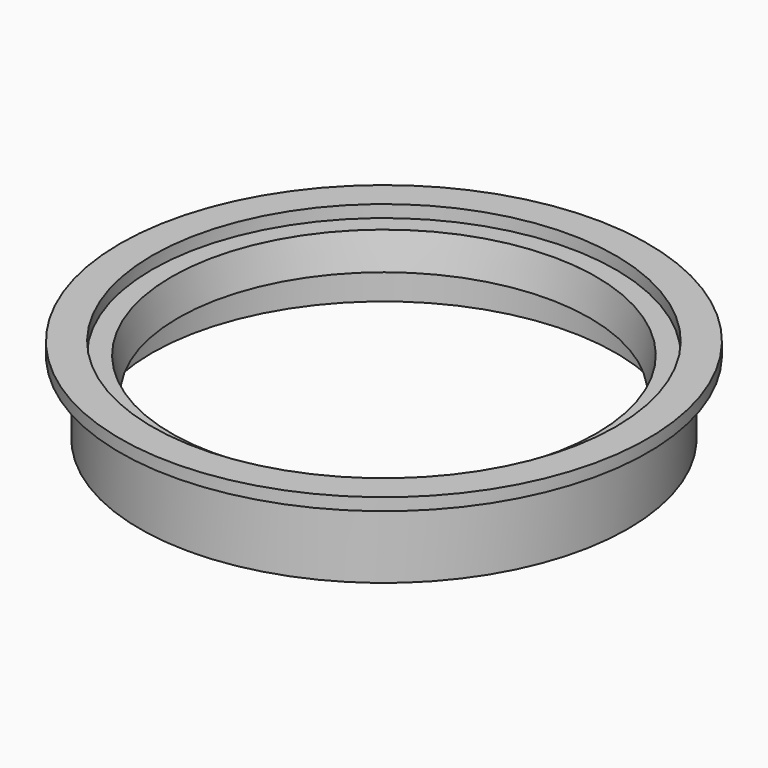
from build123d import *

# Parameters (mm, degrees)
F0_W = 1.2508329971
F0_H = 1.489882911


# Not quite as in the source:
# - ends of sketch curves that miss each other by under 0.0002 mm in the source are joined


with BuildPart() as f1:
    # F0 (on Front) → F1 (revolve)
    with BuildSketch(Plane.XZ):
        Polygon((-10.2681356725, 15.1391583099), (-10.2681356725, 15.1379262976), (-10.2489686697, 15.1379262976), (-10.2489686697, 16.4217564627), (-10.2681356725, 16.4217564627), (-13.5981356725, 16.4217564627), (-13.5981356725, 15.1391583099), (-11.5381356725, 15.1391583099), align=None)
        with Locations((-10.8935521711, 14.3929848421)):
            Rectangle(F0_W, F0_H)
        Polygon((-10.2489686697, 15.1379262976), (-10.2681356725, 15.1379262976), (-10.2681356725, 13.6480433866), (-9.4267865643, 13.6480433866), (-8.2180183381, 15.1380142197), align=None)
        Polygon((-11.5189686697, 13.6480433866), (-11.5189686697, 15.1379262976), (-11.5381356725, 15.1379262976), (-11.5381356725, 7.4834876391), (-10.2681356725, 7.4834876391), (-10.2681356725, 13.6480433866), align=None)
    revolve(axis=Axis((13.9018643275, 0, 9.1203928459), (0, 0, -1)))


with BuildPart() as f1b:
    # F0 (on Front) → F1, piece 2 (revolve)
    with BuildSketch(Plane.XZ):
        Polygon((-8.2171776903, 13.6480433866), (-9.4267865643, 13.6480433866), (-8.4628937766, 11.5783596411), (-7.5445417837, 11.5783596411), (-8.2171776903, 15.1335709829), align=None)
        Polygon((-8.2178459705, 15.1371031726), (-9.4267865643, 13.6480433866), (-8.2171776903, 13.6480433866), (-8.2171776903, 15.1335709829), align=None)
    revolve(axis=Axis((13.9018643275, 0, 9.1203928459), (0, 0, -1)))


solid = Compound([f1.part, f1b.part])
